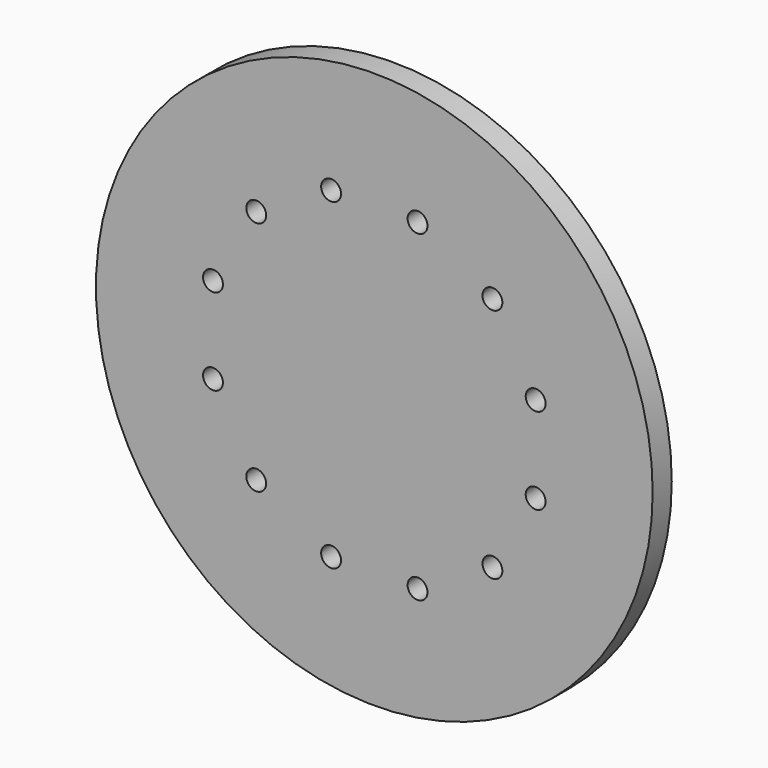
from build123d import *

# Parameters (mm, degrees)
F0_R            = 70
F1_DEPTH        = 3
F2_R            = 2.5
F3_DEPTH        = 12.5
F3_COPIES_COUNT = 12


# Not quite as in the source:
# - a pattern or mirror of a feature is missing from the dataset's text; its kind, count and spacing are read off the source's solid


with BuildPart() as f1:
    # F0 (on Front) → F1 (new body, symmetric)
    with BuildSketch(Plane.XZ):
        Circle(F0_R)
    extrude(amount=F1_DEPTH, both=True)

    # F2 (on Front) → F3 (cut, symmetric)
    with BuildSketch(Plane.XZ):
        with Locations((10.8703998943, 40.5688847041)):
            Circle(F2_R)
    f3 = extrude(amount=F3_DEPTH, both=True, mode=Mode.SUBTRACT)

    # F3_copies: F3 ×12 about axis
    f3_copies_axis = Axis((0, 0, 0), (0, 1, 0))
    for i in range(1, F3_COPIES_COUNT):
        add(f3.rotate(f3_copies_axis, i * 360 / F3_COPIES_COUNT), mode=Mode.SUBTRACT)


solid = f1.part
